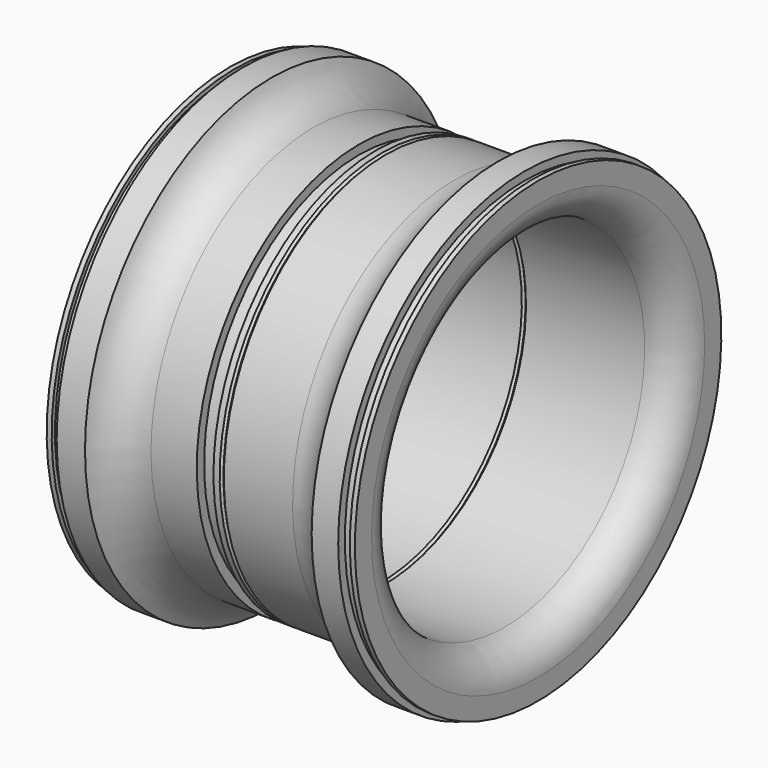
from build123d import *


# Not quite as in the source:
# - ends of sketch curves that miss each other by under 0.0002 mm in the source are joined


with BuildPart() as f1:
    # F0 (on Front) → F1 (revolve)
    with BuildSketch(Plane.XZ):
        with BuildLine():
            Line((4, 21), (18.25, 21))
            Line((18.25, 21), (18.5, 21.25))
            Line((18.5, 21.25), (18.75, 21))
            Line((18.75, 21), (33, 21))
            ThreePointArc((33, 21), (35.8284271247, 22.1715728753), (37, 25))
            Line((37, 25), (37, 27.5))
            Line((37, 27.5), (36.4, 27.5))
            Line((36.4, 27.5), (36.4, 27))
            Line((36.4, 27), (35.4, 27))
            Line((35.4, 27), (35.4, 28))
            Line((35.4, 28), (32.214393, 28))
            ThreePointArc((32.214393, 28), (30.1823197382, 25.3531604535), (26.99975, 24.35))
            Line((26.99975, 24.35), (18.75, 24.35))
            Line((18.75, 24.35), (18.5, 24.1))
            Line((18.5, 24.1), (18.25, 24.35))
            Line((18.25, 24.35), (17.5, 24.35))
            Line((17.5, 24.35), (17.5, 23.25))
            Line((17.5, 23.25), (15.5, 23.25))
            Line((15.5, 23.25), (15.5, 24.35))
            Line((15.5, 24.35), (10.00025, 24.35))
            ThreePointArc((10.00025, 24.35), (6.9048905694, 25.3595695979), (5.0000000057, 28.0000000018))
            Line((5.0000000057, 28.0000000018), (1.6, 28))
            Line((1.6, 28), (1.6, 27))
            Line((1.6, 27), (0.6, 27))
            Line((0.6, 27), (0.6, 27.5))
            Line((0.6, 27.5), (0, 27.5))
            Line((0, 27.5), (0, 25))
            ThreePointArc((0, 25), (1.1715728753, 22.1715728753), (4, 21))
        make_face()
    revolve(axis=Axis((18.5, 0, 0), (1, 0, 0)))


solid = f1.part
